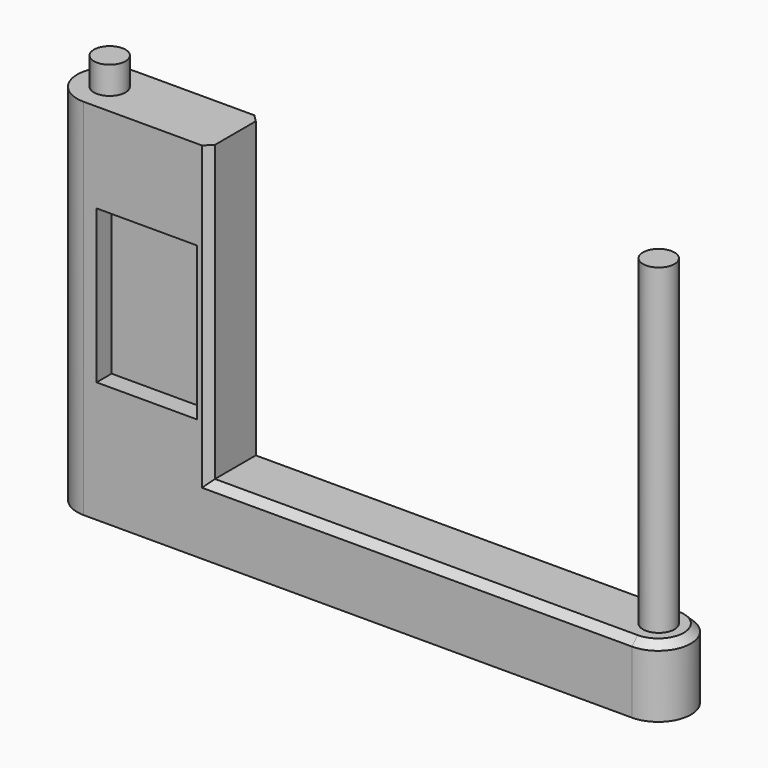
from build123d import *

# Parameters (mm, degrees)
F0_W     = 118.0431097746
F0_H     = 18.2562172413
F1_DEPTH = 19.4758269936
F0_W_2   = 35.0601822138
F2_DEPTH = 101.6
F3_W     = 28.001986444
F3_H     = 42.7611395717
F4_DEPTH = 5.2572349086
F8_R     = 4.4035732841
F9_DEPTH = 109.2703565955
F10_SIZE = 2


# Not quite as in the source:
# - a feature of the source that left no trace in its solid (it failed there, or was rolled back) is left out


with BuildPart() as f1:
    # F0 (on Top) → F1 (new body)
    with BuildSketch(Plane.XY):
        with BuildLine():
            Line((76.5516459942, 9.1281086206), (76.5516459942, -9.1281086206))
            ThreePointArc((76.5516459942, -9.1281086206), (85.6797546148, 0), (76.5516459942, 9.1281086206))
        make_face()
        with Locations((17.5300911069, 0)):
            Rectangle(F0_W, F0_H)
    extrude(amount=F1_DEPTH)

    # F0 (on Top) → F2 (join)
    with BuildSketch(Plane.XY):
        with Locations((-59.0215548873, 0)):
            Rectangle(F0_W_2, F0_H)
        with BuildLine():
            ThreePointArc((-76.5516459942, 9.1281086206), (-85.6797546148, 0), (-76.5516459942, -9.1281086206))
            Line((-76.5516459942, -9.1281086206), (-76.5516459942, 9.1281086206))
        make_face()
    extrude(amount=F2_DEPTH)

    # F3 (on face) → F4 (cut)
    with BuildSketch(Plane.XZ.offset(9.1281086206)):
        with Locations((-58.9374192059, 55.1895685494)):
            Rectangle(F3_W, F3_H)
    extrude(amount=-F4_DEPTH, mode=Mode.SUBTRACT)

    # F8 (on Top) → F9 (join)
    with BuildSketch(Plane.XY):
        with Locations((76.6932368279, 0)):
            Circle(F8_R)
        with Locations((-76.5735656023, 0)):
            Circle(F8_R)
    extrude(amount=F9_DEPTH)

    # F10
    f10_edges = [f1.edges().sort_by_distance(p)[0] for p in [
        (-41.491464, -9.128109, 60.537913),
        (17.530091, -9.128109, 19.475827),
        (-41.491464, 9.128109, 60.537913),
        (85.679755, 0, 19.475827),
        (17.530091, 9.128109, 19.475827),
    ]]
    chamfer(f10_edges, length=F10_SIZE)


solid = f1.part
